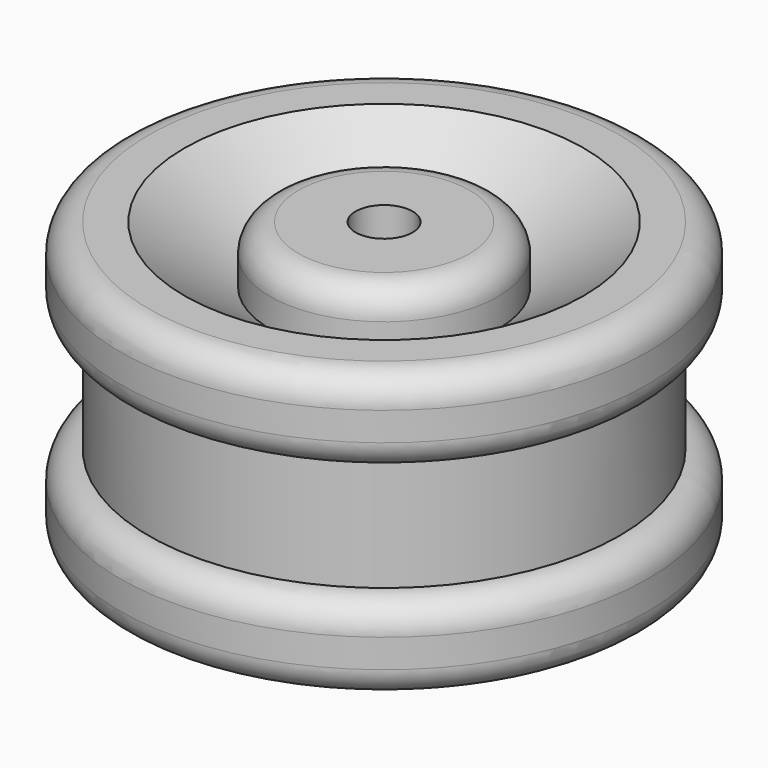
from build123d import *

# Parameters (mm, degrees)
F0_R      = 9.25
F0_R_2    = 1
F1_DEPTH  = 10
F4_R      = 7
F3_R      = 4
F8_R      = 7
F7_R      = 4
F11_R     = 4
F11_R_2   = 1
F12_DEPTH = 2
F14_R     = 9.25
F14_R_2   = 8.25
F15_DEPTH = 4
F16_R     = 0.99999


# Not quite as in the source:
# - a fillet or chamfer is up to 0.001 mm smaller than in the source, because OpenCascade refuses the exact size
# - a feature of the source that left no trace in its solid (it failed there, or was rolled back) is left out
# - a pattern or mirror of a feature is missing from the dataset's text; its kind, count and spacing are read off the source's solid


with BuildPart() as f1:
    # F0 (on Top) → F1 (new body)
    with BuildSketch(Plane.XY):
        Circle(F0_R)
        Circle(F0_R_2, mode=Mode.SUBTRACT)
    extrude(amount=F1_DEPTH)

    # F4 (on face) → F5 section 0
    with BuildSketch(Plane.XY.offset(10)):
        Circle(F4_R)
    # F3 (on offset) → F5 section 1
    with BuildSketch(Plane.XY.offset(8)):
        Circle(F3_R)
    loft(mode=Mode.SUBTRACT)

    # F8 (on face) → F9 section 0
    with BuildSketch(Plane.XY):
        Circle(F8_R)
    # F7 (on offset) → F9 section 1
    with BuildSketch(Plane.XY.offset(2)):
        Circle(F7_R)
    loft(mode=Mode.SUBTRACT)

    # F11 (on face) → F12 (join, through all)
    with BuildSketch(Plane.XY):
        Circle(F11_R)
        Circle(F11_R_2, mode=Mode.SUBTRACT)
    f12 = extrude(amount=F12_DEPTH)

    # F12_copies: F12 across plane
    add(f12.mirror(Plane.XY.offset(5)))

    # F14 (on offset) → F15 (cut)
    with BuildSketch(Plane.XY.offset(3)):
        Circle(F14_R)
        Circle(F14_R_2, mode=Mode.SUBTRACT)
    extrude(amount=F15_DEPTH, mode=Mode.SUBTRACT)

    # F16 (radius 1 in the source; OpenCascade refuses exactly that, so slightly less here)
    f16_edges = [f1.edges().sort_by_distance(p)[0] for p in [
        (-4, 0, 0),
        (-9.25, 0, 10),
        (-9.25, 0, 0),
        (-9.25, 0, 7),
        (-9.25, 0, 3),
        (-4, 0, 10),
    ]]
    fillet(f16_edges, radius=F16_R)


solid = f1.part
